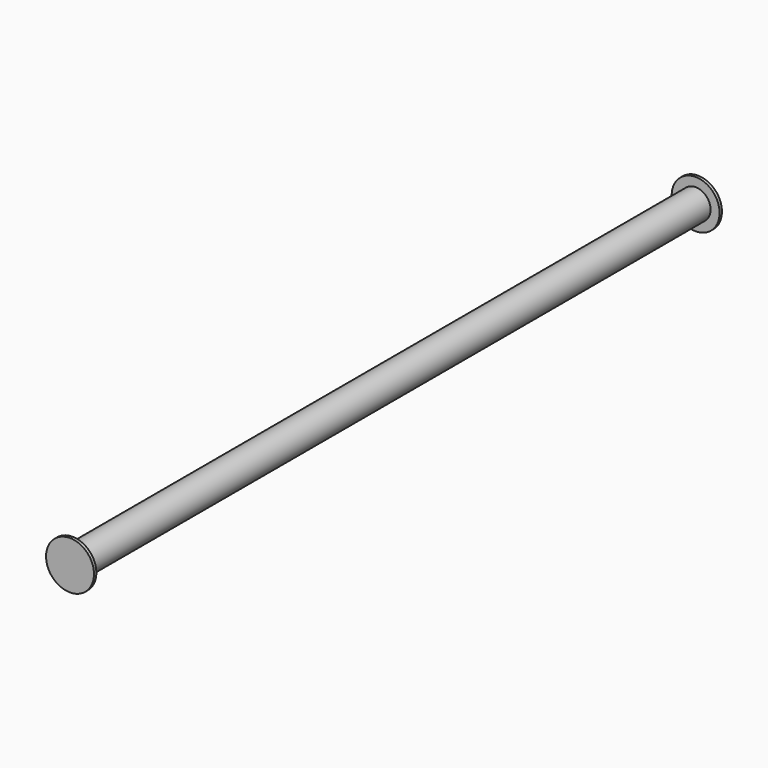
from build123d import *

# Parameters (mm, degrees)
F0_R     = 0.127
F1_DEPTH = 6.604
F2_R     = 0.2032
F2_R_2   = 0.127
F3_DEPTH = 0.0254
F4_R     = 0.2030483618
F4_R_2   = 0.127
F5_DEPTH = 0.0254


with BuildPart() as f1:
    # F0 (on Front) → F1 (new body)
    with BuildSketch(Plane.XZ):
        Circle(F0_R)
    extrude(amount=F1_DEPTH)

    # F2 (on face) → F3 (join)
    with BuildSketch(Plane.XZ.offset(6.604)):
        Circle(F2_R)
        Circle(F2_R_2, mode=Mode.SUBTRACT)
        Circle(F2_R_2)
    extrude(amount=F3_DEPTH)

    # F4 (on face) → F5 (join)
    with BuildSketch(Plane(origin=(0, 0, 0), x_dir=(-1, 0, 0), z_dir=(0, 1, 0))):
        Circle(F4_R)
        Circle(F4_R_2, mode=Mode.SUBTRACT)
        Circle(F4_R_2)
    extrude(amount=F5_DEPTH)


solid = f1.part
